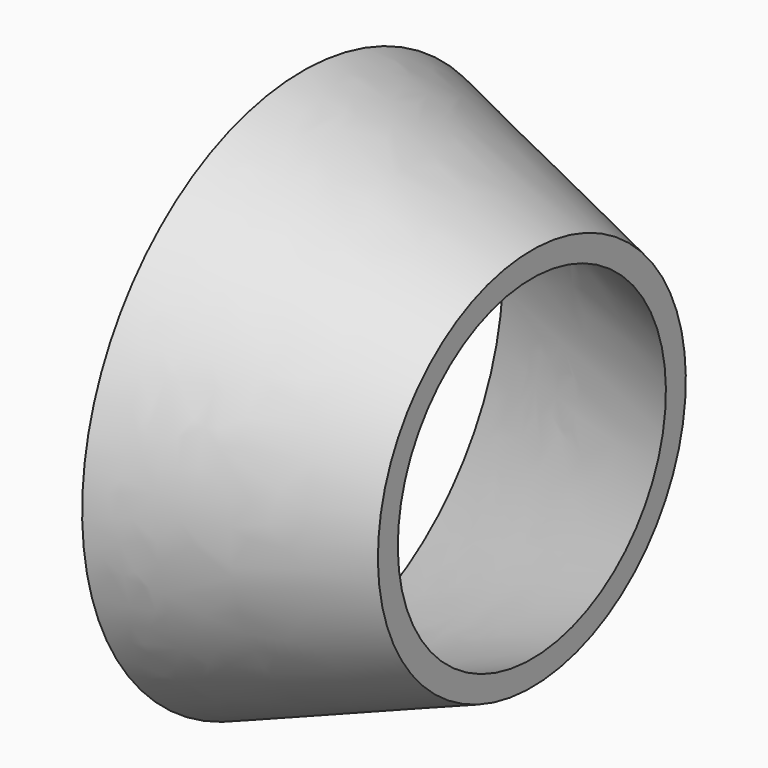
from build123d import *

# Parameters (mm, degrees)
F1_DEPTH  = 7.5
F2_W      = 2.6
F2_H      = 4.75
F0_R      = 18.75
F4_DEPTH  = 2.375
F8_R      = 4
F9_W      = 7.5
F9_H      = 50
F10_DEPTH = 86


# Not quite as in the source:
# - a feature names something its author has since deleted; it is built from what else it names


with BuildPart() as f1:
    # F0 (on Right) → F1 (new body)
    with BuildSketch(Plane.YZ):
        with BuildLine():
            Line((-27.5, -30.8578620553), (-27.5, 35))
            Line((-27.5, 35), (-35, 35))
            Line((-35, 35), (-35, -33.3578620553))
            ThreePointArc((-35, -33.3578620553), (-32.0710678119, -40.4289298672), (-25, -43.3578620553))
            Line((-25, -43.3578620553), (25, -43.3578620553))
            ThreePointArc((25, -43.3578620553), (32.0710678119, -40.4289298672), (35, -33.3578620553))
            Line((35, -33.3578620553), (35, 35))
            Line((35, 35), (27.5, 35))
            Line((27.5, 35), (27.5, -30.8578620553))
            ThreePointArc((27.5, -30.8578620553), (26.0355339059, -34.3933959612), (22.5, -35.8578620553))
            Line((22.5, -35.8578620553), (-22.5, -35.8578620553))
            ThreePointArc((-22.5, -35.8578620553), (-26.0355339059, -34.3933959612), (-27.5, -30.8578620553))
        make_face()
    extrude(amount=F1_DEPTH)

    # F3: sweep along a path in F0
    with BuildLine(Plane.YZ) as f3_path:
        Line((27.5, 35), (27.5, -30.8578620553))
        ThreePointArc((27.5, -30.8578620553), (26.0355339059, -34.3933959612), (22.5, -35.8578620553))
        Line((22.5, -35.8578620553), (-22.5, -35.8578620553))
        ThreePointArc((-22.5, -35.8578620553), (-26.0355339059, -34.3933959612), (-27.5, -30.8578620553))
        Line((-27.5, -30.8578620553), (-27.5, 35))
    # F2 (on face) → F3 (sweep, cut)
    with BuildSketch(Plane.XY.offset(35)):
        with Locations((3.675, 29.875)):
            Rectangle(F2_W, F2_H)
    sweep(path=f3_path.line, mode=Mode.SUBTRACT)

    # F0 (on Right) → F4 (join)
    with BuildSketch(Plane.YZ):
        with BuildLine():
            Line((27.5, 35), (-27.5, 35))
            Line((-27.5, 35), (-27.5, -30.8578620553))
            ThreePointArc((-27.5, -30.8578620553), (-26.0355339059, -34.3933959612), (-22.5, -35.8578620553))
            Line((-22.5, -35.8578620553), (22.5, -35.8578620553))
            ThreePointArc((22.5, -35.8578620553), (26.0355339059, -34.3933959612), (27.5, -30.8578620553))
            Line((27.5, -30.8578620553), (27.5, 35))
        make_face()
        with Locations((2, 3)):
            Circle(F0_R, mode=Mode.SUBTRACT)
    extrude(amount=F4_DEPTH)

    # F6 (on offset) → F7 (revolve)
    with BuildSketch(Plane.XY.offset(1)):
        Polygon((0, 22), (0, 25), (-27.5, 35), (-27.5, 32), align=None)
    revolve(axis=Axis((0, 2, 3), (1, 0, 0)))

    # F8
    f8_edges = [f1.edges().sort_by_distance(p)[0] for p in [
        (6.2375, -27.5, 35),
        (6.2375, 27.5, 35),
    ]]
    fillet(f8_edges, radius=F8_R)

    # F9 (on face) → F10 (cut)
    with BuildSketch(Plane(origin=(0, 0, -43.3578620553), x_dir=(1, 0, 0), z_dir=(0, 0, -1))):
        Polygon((0, -25), (0, -46.4285723865), (9.4410963356, -46.4285723865), (9.4410963356, 44.8143593967), (0, 44.8143593967), (0, 25), (7.5, 25), (7.5, -25), align=None)
        with Locations((3.75, 0)):
            Rectangle(F9_W, F9_H)
    extrude(amount=-F10_DEPTH, mode=Mode.SUBTRACT)


solid = f1.part
